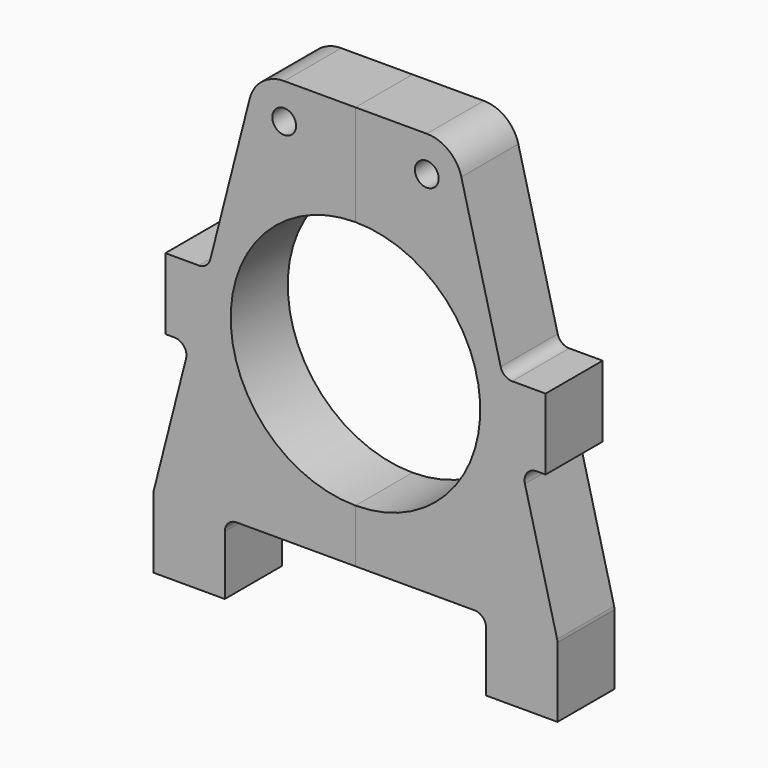
from build123d import *
from build123d import SkipClean  # not in build123d's __all__

# Parameters (mm, degrees)
F0_R     = 5
F1_DEPTH = 15
F2_R     = 5


with BuildPart() as f1:
    # F0 (on Front) → F1 (new body, symmetric)
    with BuildSketch(Plane.XZ):
        with BuildLine():
            Line((-85, 30), (-85, 0))
            Line((-85, 0), (-55, 0))
            Line((-55, 0), (-55, 30))
            Line((-55, 30), (0, 30))
            Line((0, 30), (0, 52.5))
            ThreePointArc((0, 52.5), (-52.5, 105), (0, 157.5))
            Line((0, 157.5), (0, 200))
            Line((0, 200), (-30, 200))
            ThreePointArc((-30, 200), (-39.2035469986, 196.8446073234), (-44.5349866907, 188.7059630193))
            Line((-44.5349866907, 188.7059630193), (-62.0528395496, 120))
            Line((-62.0528395496, 120), (-80, 120))
            Line((-80, 120), (-80, 90))
            Line((-80, 90), (-69.7018930331, 90))
            Line((-69.7018930331, 90), (-85, 30))
        make_face()
        with Locations((-30, 185)):
            Circle(F0_R, mode=Mode.SUBTRACT)
    extrude(amount=F1_DEPTH, both=True)

    # F2
    f2_edges = [f1.edges().sort_by_distance(p)[0] for p in [
        (-69.701893, 0, 90),
        (-62.05284, 0, 120),
        (-85, 0, 30),
        (-55, 0, 30),
    ]]
    fillet(f2_edges, radius=F2_R)

    # F3: F1 across plane


with BuildPart() as f1_1:
    add(f1.part, clean=False)
    with SkipClean():  # cleaning this boolean's faces spoils the solid; the shape is the same uncleaned
        add(f1.part.mirror(Plane.YZ), clean=False)


solid = f1_1.part
